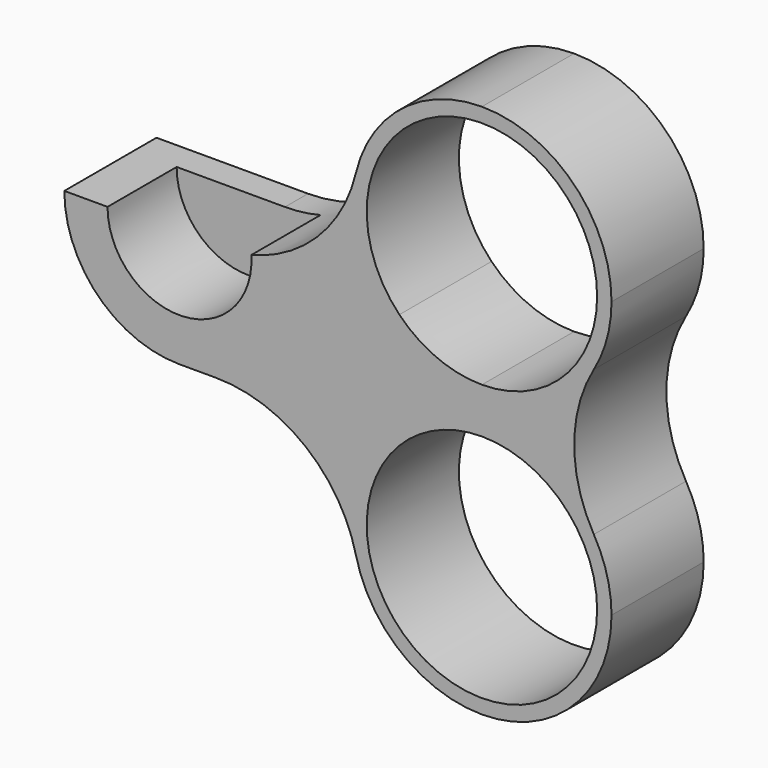
from build123d import *

# Parameters (mm, degrees)
F1_DEPTH = 4
F2_R     = 5
F3_R     = 3.99999
F4_DEPTH = 3


# Not quite as in the source:
# - a fillet or chamfer is up to 0.001 mm smaller than in the source, because OpenCascade refuses the exact size


with BuildPart() as f1:
    # F0 (on Front) → F1 (new body)
    with BuildSketch(Plane.XZ):
        with BuildLine():
            ThreePointArc((4.5, 0), (3.1819805153, 3.1819805153), (0, 4.5))
            ThreePointArc((0, 4.5), (-3.1819805153, 3.1819805153), (-4.5, 0))
            ThreePointArc((-4.5, 0), (-4.2507756145, -1.4767893131), (-3.5307081443, -2.79))
            Line((-3.5307081443, -2.79), (-2.8663391286, -2.79))
            ThreePointArc((-2.8663391286, -2.79), (-1.5057628442, 3.7057628442), (4, 0))
            ThreePointArc((4, 0), (2.8284271247, -2.8284271247), (0, -4))
            Line((0, -4), (0, -4.5))
            ThreePointArc((0, -4.5), (2.2405062847, -3.9025801194), (3.8861134595, -2.2689473726))
            ThreePointArc((3.8861134595, -2.2689473726), (4.3438180537, -1.1752636794), (4.5, 0))
        make_face()
        with BuildLine():
            ThreePointArc((4.5, -9.58), (4.3438180596, -8.4047363422), (3.886113482, -7.3110526659))
            ThreePointArc((3.886113482, -7.3110526659), (2.240506304, -5.6774198917), (0, -5.08))
            Line((0, -5.08), (0, -5.58))
            ThreePointArc((0, -5.58), (2.8284271247, -6.7515728753), (4, -9.58))
            ThreePointArc((4, -9.58), (-1.5057628442, -13.2857628442), (-2.8663391286, -6.79))
            Line((-2.8663391286, -6.79), (-3.5307081443, -6.79))
            ThreePointArc((-3.5307081443, -6.79), (-4.2507756145, -8.1032106869), (-4.5, -9.58))
            ThreePointArc((-4.5, -9.58), (-3.1819805153, -12.7619805153), (0, -14.08))
            ThreePointArc((0, -14.08), (3.1819805153, -12.7619805153), (4.5, -9.58))
        make_face()
        with BuildLine():
            Line((-2.8663391286, -2.79), (-3.5307081443, -2.79))
            ThreePointArc((-3.5307081443, -2.79), (-1.9615045246, -4.05), (0, -4.5))
            Line((0, -4.5), (0, -4))
            ThreePointArc((0, -4), (-1.5556349186, -3.6851051545), (-2.8663391286, -2.79))
        make_face()
        with BuildLine():
            ThreePointArc((0, -5.08), (-1.9615045246, -5.53), (-3.5307081443, -6.79))
            Line((-3.5307081443, -6.79), (-2.8663391286, -6.79))
            ThreePointArc((-2.8663391286, -6.79), (-1.5556349186, -5.8948948455), (0, -5.58))
            Line((0, -5.58), (0, -5.08))
        make_face()
        with BuildLine():
            Line((-3.5307081443, -2.79), (-4.5, -2.79))
            Line((-4.5, -2.79), (-4.5, -6.79))
            Line((-4.5, -6.79), (-3.5307081443, -6.79))
            ThreePointArc((-3.5307081443, -6.79), (-1.9615045246, -5.53), (0, -5.08))
            Line((0, -5.08), (0, -4.5))
            ThreePointArc((0, -4.5), (-1.9615045246, -4.05), (-3.5307081443, -2.79))
        make_face()
        with BuildLine():
            ThreePointArc((-3.5307081443, -2.79), (-4.2507756145, -1.4767893131), (-4.5, 0))
            Line((-4.5, 0), (-4.5, -2.79))
            Line((-4.5, -2.79), (-3.5307081443, -2.79))
        make_face()
        with BuildLine():
            Line((-3.5307081443, -6.79), (-4.5, -6.79))
            Line((-4.5, -6.79), (-4.5, -9.58))
            ThreePointArc((-4.5, -9.58), (-4.2507756145, -8.1032106869), (-3.5307081443, -6.79))
        make_face()
        with BuildLine():
            Line((-4.5, -6.79), (-4.5, -2.79))
            Line((-4.5, -2.79), (-8, -2.79))
            ThreePointArc((-8, -2.79), (-10.5, -5.29), (-13, -2.79))
            Line((-13, -2.79), (-14.5, -2.79))
            Line((-14.5, -2.79), (-14.5, -6.79))
            Line((-14.5, -6.79), (-4.5, -6.79))
        make_face()
        with BuildLine():
            ThreePointArc((-13, -2.79), (-10.5, -5.29), (-8, -2.79))
            Line((-8, -2.79), (-13, -2.79))
        make_face()
        with BuildLine():
            ThreePointArc((3.886113482, -7.3110526659), (3.2040173086, -4.7900000223), (3.8861134595, -2.2689473726))
            ThreePointArc((3.8861134595, -2.2689473726), (2.2405062847, -3.9025801194), (0, -4.5))
            Line((0, -4.5), (0, -5.08))
            ThreePointArc((0, -5.08), (2.240506304, -5.6774198917), (3.886113482, -7.3110526659))
        make_face()
    extrude(amount=-F1_DEPTH)

    # F2
    f2_edges = [f1.edges().sort_by_distance(p)[0] for p in [
        (-4.5, 2, -2.79),
        (-4.5, 2, -6.79),
    ]]
    fillet(f2_edges, radius=F2_R)

    # F3 (radius 4 in the source; OpenCascade refuses exactly that, so slightly less here)
    f3_edges = [f1.edges().sort_by_distance(p)[0] for p in [
        (-14.5, 2, -6.79),
    ]]
    fillet(f3_edges, radius=F3_R)

    # F0 (on Front) → F4 (cut)
    with BuildSketch(Plane.XZ):
        with BuildLine():
            ThreePointArc((-13, -2.79), (-10.5, -5.29), (-8, -2.79))
            Line((-8, -2.79), (-13, -2.79))
        make_face()
        with BuildLine():
            Line((-13, -2.79), (-8, -2.79))
            ThreePointArc((-8, -2.79), (-10.5, -0.29), (-13, -2.79))
        make_face()
    extrude(amount=-F4_DEPTH, mode=Mode.SUBTRACT)


solid = f1.part
